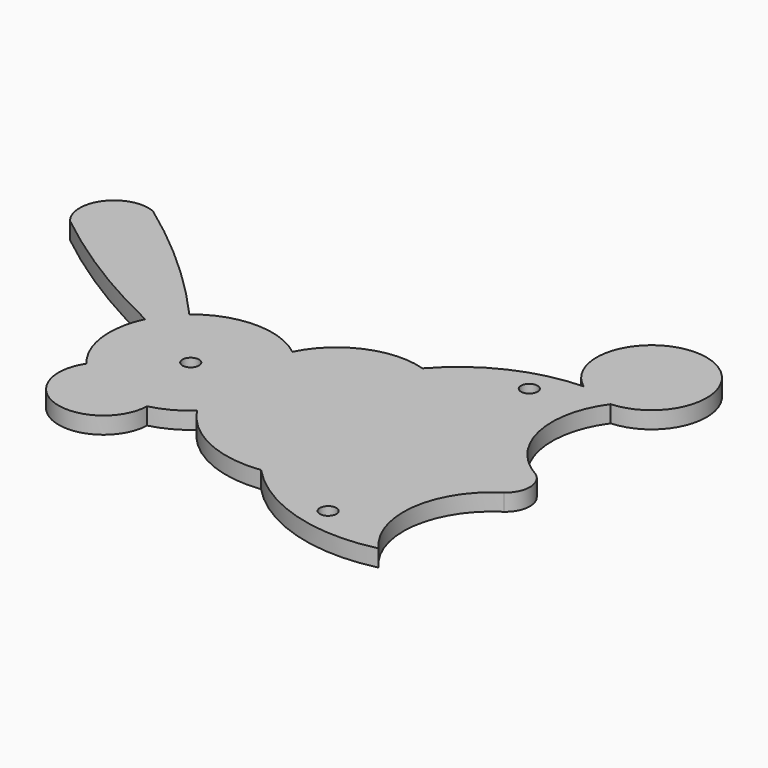
from build123d import *

# Parameters (mm, degrees)
F1_R     = 0.975
F1_R_2   = 5.495
F2_DEPTH = 2


# Not quite as in the source:
# - the program builds the solid bodies; features that only make, move or delete a surface that nothing else refers to are left out


with BuildPart() as f2:
    # F1 (on Top) → F2 (new body)
    with BuildSketch(Plane.XY):
        with BuildLine():
            ThreePointArc((8.3461548541, 12.451567302), (1.7252198574, 12.0948349613), (-3.0867358283, 7.5331334509))
            ThreePointArc((-3.0867358283, 7.5331334509), (-9.1504459177, 9.6196614304), (-15.1782928372, 7.431685066))
            ThreePointArc((-15.1782928372, 7.431685066), (-22.5381757879, 14.8578874844), (-30.6692253798, 21.4307401329))
            ThreePointArc((-30.6692253798, 21.4307401329), (-35.5250947404, 20.1584087851), (-35.4319922626, 15.1394819841))
            ThreePointArc((-35.4319922626, 15.1394819841), (-26.9109452732, 9.1280444677), (-17.7545223506, 4.1374991998))
            ThreePointArc((-17.7545223506, 4.1374991998), (-18.6125164693, -1.2164521529), (-16.4388114376, -6.1839420049))
            ThreePointArc((-16.4388114376, -6.1839420049), (-13.6846503599, -14.1883393203), (-6.7486233515, -9.3357823691))
            ThreePointArc((-6.7486233515, -9.3357823691), (-4.5490625181, -8.4916373097), (-2.6206436977, -7.1381789267))
            ThreePointArc((-2.6206436977, -7.1381789267), (2.5909813664, -11.6392406956), (9.3949967995, -12.7003565431))
            ThreePointArc((9.3949967995, -12.7003565431), (17.7901975829, -17.882711986), (27.6524089277, -18.1528814137))
            ThreePointArc((27.6524089277, -18.1528814137), (24.9662444476, -9.7026669711), (29.7177772104, -2.2163768254))
            ThreePointArc((29.7177772104, -2.2163768254), (30.8881367766, 0.1144698658), (29.7177772104, 2.4453165571))
            ThreePointArc((29.7177772104, 2.4453165571), (24.594325339, 9.3144076758), (26.3560396261, 17.700737901))
            ThreePointArc((26.3560396261, 17.700737901), (27.8220537541, 30.4194435664), (22.2002219007, 18.9168491704))
            ThreePointArc((22.2002219007, 18.9168491704), (14.5953140013, 17.1367848208), (8.3461548541, 12.451567302))
        make_face()
        with BuildLine():
            Line((-17.6755707347, -0.4939858073), (-12.0034380316, -0.4939858073))
            ThreePointArc((-12.0034380316, -0.4939858073), (-10.5336675739, -2.589890275), (-7.9799964747, -2.7682288675))
            Line((-7.9799964747, -2.7682288675), (-5.2005199999, -7.702828149))
            ThreePointArc((-5.2005199999, -7.702828149), (-5.9901385216, -8.0511163546), (-6.810625891, -8.3187029026))
            ThreePointArc((-6.810625891, -8.3187029026), (-7.2968984625, -8.4404428952), (-7.7895048721, -8.5332898913))
            ThreePointArc((-7.7895048721, -8.5332898913), (-13.3753397984, -13.2373782399), (-15.1250045058, -6.1473378715))
            ThreePointArc((-15.1250045058, -6.1473378715), (-15.4687321672, -5.7824640106), (-15.7903406401, -5.3979518136))
            ThreePointArc((-15.7903406401, -5.3979518136), (-17.1156764189, -3.0930980197), (-17.6755707347, -0.4939858073))
        make_face(mode=Mode.SUBTRACT)
        with Locations((-9.069736782, 0)):
            Circle(F1_R, mode=Mode.SUBTRACT)
        with Locations((19.3387361329, -15.2233078331)):
            Circle(F1_R, mode=Mode.SUBTRACT)
        with BuildLine():
            ThreePointArc((20.3872606575, 17.7804109262), (22.7170872685, 17.9218257414), (25.0456576674, 17.7610461256))
            ThreePointArc((25.0456576674, 17.7610461256), (25.1091906486, 17.7523846185), (25.172692422, 17.7434972003))
            ThreePointArc((25.172692422, 17.7434972003), (23.684740061, 8.8128379715), (29.166954709, 1.6075621931))
            ThreePointArc((29.166954709, 1.6075621931), (29.8880875558, 0.1007714549), (29.1453733807, -1.3954994316))
            ThreePointArc((29.1453733807, -1.3954994316), (24.1127403048, -8.7463736841), (25.8509191741, -17.4837349662))
            ThreePointArc((25.8509191741, -17.4837349662), (23.5178476173, -17.6742786032), (21.1797885868, -17.5602183711))
            ThreePointArc((21.1797885868, -17.5602183711), (20.0605128424, -12.3371922115), (16.6143622853, -16.4184698048))
            ThreePointArc((16.6143622853, -16.4184698048), (12.9131993659, -14.4284100321), (9.7748074556, -11.6338723113))
            ThreePointArc((9.7748074556, -11.6338723113), (2.6662624957, -10.5651214915), (-2.4218244994, -5.4872271944))
            ThreePointArc((-2.4218244994, -5.4872271944), (-3.341520275, -6.4414234179), (-4.3966137229, -7.2433639198))
            Line((-4.3966137229, -7.2433639198), (-7.1815796443, -2.2990188393))
            ThreePointArc((-7.1815796443, -2.2990188393), (-6.094920293, 0.0330432552), (-7.2331126554, 2.3403924495))
            Line((-7.2331126554, 2.3403924495), (-4.4863168152, 7.3004562466))
            ThreePointArc((-4.4863168152, 7.3004562466), (-3.5431905745, 6.6152616741), (-2.7011412367, 5.8090783073))
            ThreePointArc((-2.7011412367, 5.8090783073), (1.7884096787, 11.0249893996), (8.6656284498, 11.2812274136))
            ThreePointArc((8.6656284498, 11.2812274136), (11.9172089396, 14.3848906615), (15.8355289242, 16.5876774731))
            ThreePointArc((15.8355289242, 16.5876774731), (19.3270471679, 12.5448488398), (20.3872606575, 17.7804109262))
        make_face(mode=Mode.SUBTRACT)
        with BuildLine():
            ThreePointArc((-16.3638620166, 4.5934885503), (-26.0025688441, 9.741867589), (-34.9414590553, 16.0273045526))
            ThreePointArc((-34.9414590553, 16.0273045526), (-34.7398034138, 19.6908643856), (-31.1758954498, 20.5631577259))
            ThreePointArc((-31.1758954498, 20.5631577259), (-22.796689347, 13.7414479433), (-15.2552633126, 6.0036373591))
            ThreePointArc((-15.2552633126, 6.0036373591), (-10.598818784, 8.4832958354), (-5.3696469446, 7.7854823354))
            Line((-5.3696469446, 7.7854823354), (-8.119843394, 2.8192778422))
            ThreePointArc((-8.119843394, 2.8192778422), (-10.5540740424, 2.5782489983), (-11.9848002521, 0.5941632478))
            Line((-11.9848002521, 0.5941632478), (-17.6692350252, 0.5941632478))
            ThreePointArc((-17.6692350252, 0.5941632478), (-17.2642756667, 2.67468362), (-16.3638620166, 4.5934885503))
        make_face(mode=Mode.SUBTRACT)
        with Locations((18.5729401514, 15.4226861541)):
            Circle(F1_R, mode=Mode.SUBTRACT)
        with Locations((25.9979280814, 24.1858578784)):
            Circle(F1_R_2, mode=Mode.SUBTRACT)
        with BuildLine():
            ThreePointArc((25.172692422, 17.7434972003), (25.1091317315, 17.7519581241), (25.0456576674, 17.7610461256))
            ThreePointArc((25.0456576674, 17.7610461256), (22.7170872685, 17.9218257414), (20.3872606575, 17.7804109262))
            ThreePointArc((20.3872606575, 17.7804109262), (19.3270471679, 12.5448488398), (15.8355289242, 16.5876774731))
            ThreePointArc((15.8355289242, 16.5876774731), (11.9172089396, 14.3848906615), (8.6656284498, 11.2812274136))
            ThreePointArc((8.6656284498, 11.2812274136), (1.7884096787, 11.0249893996), (-2.7011412367, 5.8090783073))
            ThreePointArc((-2.7011412367, 5.8090783073), (-3.5431905745, 6.6152616741), (-4.4863168152, 7.3004562466))
            Line((-4.4863168152, 7.3004562466), (-7.2331126554, 2.3403924495))
            ThreePointArc((-7.2331126554, 2.3403924495), (-6.094920293, 0.0330432552), (-7.1815796443, -2.2990188393))
            Line((-7.1815796443, -2.2990188393), (-4.3966137229, -7.2433639198))
            ThreePointArc((-4.3966137229, -7.2433639198), (-3.341520275, -6.4414234179), (-2.4218244994, -5.4872271944))
            ThreePointArc((-2.4218244994, -5.4872271944), (2.6662624957, -10.5651214915), (9.7748074556, -11.6338723113))
            ThreePointArc((9.7748074556, -11.6338723113), (12.9131993659, -14.4284100321), (16.6143622853, -16.4184698048))
            ThreePointArc((16.6143622853, -16.4184698048), (20.0605128424, -12.3371922115), (21.1797885868, -17.5602183711))
            ThreePointArc((21.1797885868, -17.5602183711), (23.5178476173, -17.6742786032), (25.8509191741, -17.4837349662))
            ThreePointArc((25.8509191741, -17.4837349662), (24.1127403048, -8.7463736841), (29.1453733807, -1.3954994316))
            ThreePointArc((29.1453733807, -1.3954994316), (29.8880875558, 0.1007714549), (29.166954709, 1.6075621931))
            ThreePointArc((29.166954709, 1.6075621931), (23.684740061, 8.8128379715), (25.172692422, 17.7434972003))
        make_face()
        with BuildLine():
            ThreePointArc((-31.1758954498, 20.5631577259), (-34.7398034138, 19.6908643856), (-34.9414590553, 16.0273045526))
            ThreePointArc((-34.9414590553, 16.0273045526), (-26.0025688441, 9.741867589), (-16.3638620166, 4.5934885503))
            ThreePointArc((-16.3638620166, 4.5934885503), (-17.2642756667, 2.67468362), (-17.6692350252, 0.5941632478))
            Line((-17.6692350252, 0.5941632478), (-11.9848002521, 0.5941632478))
            ThreePointArc((-11.9848002521, 0.5941632478), (-10.5540740424, 2.5782489983), (-8.119843394, 2.8192778422))
            Line((-8.119843394, 2.8192778422), (-5.3696469446, 7.7854823354))
            ThreePointArc((-5.3696469446, 7.7854823354), (-10.598818784, 8.4832958354), (-15.2552633126, 6.0036373591))
            ThreePointArc((-15.2552633126, 6.0036373591), (-22.796689347, 13.7414479433), (-31.1758954498, 20.5631577259))
        make_face()
        with BuildLine():
            ThreePointArc((-7.9799964747, -2.7682288675), (-10.5336675739, -2.589890275), (-12.0034380316, -0.4939858073))
            Line((-12.0034380316, -0.4939858073), (-17.6755707347, -0.4939858073))
            ThreePointArc((-17.6755707347, -0.4939858073), (-17.1156764189, -3.0930980197), (-15.7903406401, -5.3979518136))
            ThreePointArc((-15.7903406401, -5.3979518136), (-15.4687321672, -5.7824640106), (-15.1250045058, -6.1473378715))
            ThreePointArc((-15.1250045058, -6.1473378715), (-13.3753397984, -13.2373782399), (-7.7895048721, -8.5332898913))
            ThreePointArc((-7.7895048721, -8.5332898913), (-7.2968984625, -8.4404428952), (-6.810625891, -8.3187029026))
            ThreePointArc((-6.810625891, -8.3187029026), (-5.9901385216, -8.0511163546), (-5.2005199999, -7.702828149))
            Line((-5.2005199999, -7.702828149), (-7.9799964747, -2.7682288675))
        make_face()
        with Locations((25.9979280814, 24.1858578784)):
            Circle(F1_R_2)
    extrude(amount=F2_DEPTH)


solid = f2.part
